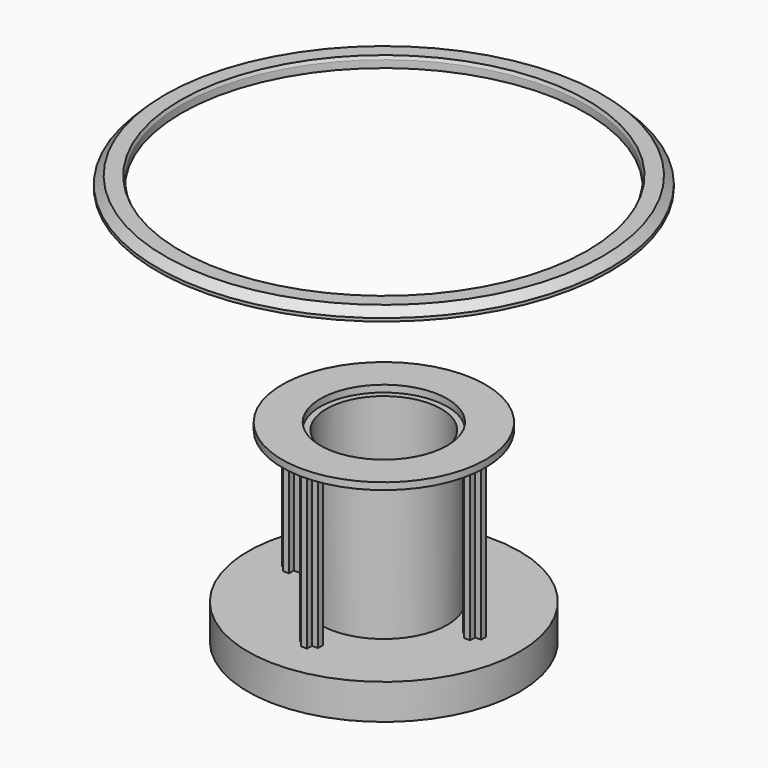
from build123d import *

# Parameters (mm, degrees)
F0_W      = 2
F0_H      = 2
F1_DEPTH  = 50
F0_R      = 21
F0_R_2    = 19
F2_DEPTH  = 50
F3_R      = 33.6748592908
F3_R_2    = 21
F4_DEPTH  = 2.286
F0_R_3    = 10.9886150932
F5_DEPTH  = 120.65
F6_R      = 75
F6_R_2    = 66.9568683552
F7_DEPTH  = 3.556
F0_R_4    = 45
F0_R_5    = 40
F11_DEPTH = 11.684
F12_DEPTH = 7.112
F13_SIZE  = 2.54
F14_SIZE  = 0.1


# Not quite as in the source:
# - a fillet or chamfer that OpenCascade refuses, or shapes differently, is made with other operations: its cross-section is extruded or revolved along the edge and cut away or added
# - the program builds the solid bodies; features that only make, move or delete a surface that nothing else refers to are left out


with BuildPart() as f1:
    # F0 (on Top) → F1 (new body)
    with BuildSketch(Plane.XY):
        with Locations((-2, 30)):
            Rectangle(F0_W, F0_H)
        with Locations((0, 32)):
            Rectangle(F0_W, F0_H)
        with Locations((2, 30)):
            Rectangle(F0_W, F0_H)
        with Locations((0, 28)):
            Rectangle(F0_W, F0_H)
        with Locations((0, 30)):
            Rectangle(F0_W, F0_H)
    extrude(amount=F1_DEPTH)



with BuildPart() as f1b:
    # F0 (on Top) → F1, piece 2 (new body)
    with BuildSketch(Plane.XY):
        with Locations((32, 0)):
            Rectangle(F0_W, F0_H)
        with Locations((28, 0)):
            Rectangle(F0_W, F0_H)
        with Locations((30, -2)):
            Rectangle(F0_W, F0_H)
        with Locations((30, 2)):
            Rectangle(F0_W, F0_H)
        with Locations((30, 0)):
            Rectangle(F0_W, F0_H)
    extrude(amount=F1_DEPTH)


with BuildPart() as f1c:
    # F0 (on Top) → F1, piece 3 (new body)
    with BuildSketch(Plane.XY):
        with Locations((0, -28)):
            Rectangle(F0_W, F0_H)
        with Locations((2, -30)):
            Rectangle(F0_W, F0_H)
        with Locations((-2, -30)):
            Rectangle(F0_W, F0_H)
        with Locations((0, -32)):
            Rectangle(F0_W, F0_H)
        with Locations((0, -30)):
            Rectangle(F0_W, F0_H)
    extrude(amount=F1_DEPTH)


with BuildPart() as f1d:
    # F0 (on Top) → F1, piece 4 (new body)
    with BuildSketch(Plane.XY):
        with Locations((-30, 2)):
            Rectangle(F0_W, F0_H)
        with Locations((-32, 0)):
            Rectangle(F0_W, F0_H)
        with Locations((-28, 0)):
            Rectangle(F0_W, F0_H)
        with Locations((-30, -2)):
            Rectangle(F0_W, F0_H)
        with Locations((-30, 0)):
            Rectangle(F0_W, F0_H)
    extrude(amount=F1_DEPTH)


with BuildPart() as f2:
    # F0 (on Top) → F2 (new body)
    with BuildSketch(Plane.XY):
        Circle(F0_R)
        Circle(F0_R_2, mode=Mode.SUBTRACT)
    extrude(amount=F2_DEPTH)


with BuildPart() as f4:
    # F3 (on face) → F4 (new body)
    with BuildSketch(Plane.XY.offset(50)):
        Circle(F3_R)
        Circle(F3_R_2, mode=Mode.SUBTRACT)
    extrude(amount=F4_DEPTH)


with BuildPart() as f5:
    # F0 (on Top) → F5 (new body)
    with BuildSketch(Plane.XY):
        Circle(F0_R_3)
    extrude(amount=F5_DEPTH)


with BuildPart() as f7:
    # F6 (on face) → F7 (new body)
    with BuildSketch(Plane.XY.offset(120.65)):
        Circle(F6_R)
        Circle(F6_R_2, mode=Mode.SUBTRACT)
    extrude(amount=F7_DEPTH)

    # F13
    f13_edges = [f7.edges().sort_by_distance(p)[0] for p in [
        (-75, 0, 124.206),
    ]]
    chamfer(f13_edges, length=F13_SIZE)

    # F14
    f14_edges = [f7.edges().sort_by_distance(p)[0] for p in [
        (-66.956868, 0, 124.206),
    ]]
    chamfer(f14_edges, length=F14_SIZE)

    # F15: chamfer of 1 on 1 edges, made by hand

    # F15_s1 → F15_t2 (revolve, cut)
    with BuildSketch(Plane.XZ):
        Polygon((67.6639751364, 124.8131067812), (66.9568683552, 123.106), (66.9568683552, 124.106), align=None)
    revolve(axis=Axis((0, 0, 124.106), (0, 0, 1)), mode=Mode.SUBTRACT)


with BuildPart() as f11:
    # F0 (on Top) → F11 (new body)
    with BuildSketch(Plane.XY):
        Circle(F0_R_4)
        Circle(F0_R_5, mode=Mode.SUBTRACT)
    extrude(amount=-F11_DEPTH)


with BuildPart() as f1_1:
    add(f1.part)

    add(f1b.part)  # F12 merges F1b

    add(f1c.part)  # F12 merges F1c

    add(f1d.part)  # F12 merges F1d

    add(f2.part)  # F12 merges F2

    add(f11.part)  # F12 merges F11
    # F0 (on Top) → F12 (join)
    with BuildSketch(Plane.XY):
        Circle(F0_R_5)
        Polygon((-1, -29), (-1, -27), (1, -27), (1, -29), (3, -29), (3, -31), (1, -31), (1, -33), (-1, -33), (-1, -31), (-3, -31), (-3, -29), align=None, mode=Mode.SUBTRACT)
        Polygon((-29, 1), (-27, 1), (-27, -1), (-29, -1), (-29, -3), (-31, -3), (-31, -1), (-33, -1), (-33, 1), (-31, 1), (-31, 3), (-29, 3), align=None, mode=Mode.SUBTRACT)
        Circle(F0_R, mode=Mode.SUBTRACT)
        Polygon((29, -1), (27, -1), (27, 1), (29, 1), (29, 3), (31, 3), (31, 1), (33, 1), (33, -1), (31, -1), (31, -3), (29, -3), align=None, mode=Mode.SUBTRACT)
        Polygon((3, 31), (3, 29), (1, 29), (1, 27), (-1, 27), (-1, 29), (-3, 29), (-3, 31), (-1, 31), (-1, 33), (1, 33), (1, 31), align=None, mode=Mode.SUBTRACT)
    extrude(amount=-F12_DEPTH)


solid = Compound([f4.part, f7.part, f1_1.part])
